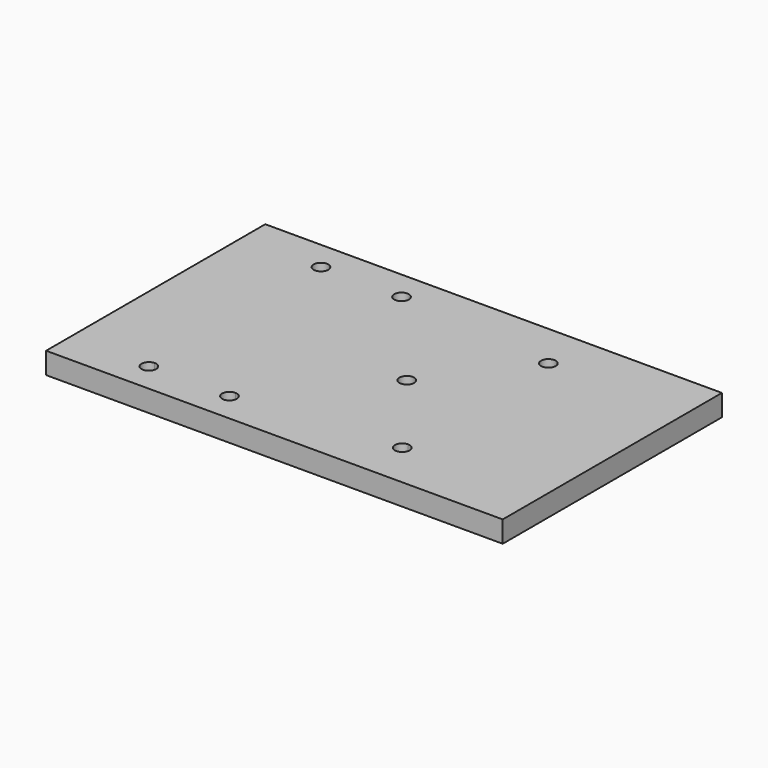
from build123d import *

# Parameters (mm, degrees)
F0_W     = 127
F0_H     = 76.2
F2_DEPTH = 5.969
F3_R     = 2.032
F4_DEPTH = 5.969


# Not quite as in the source:
# - a variable given as a bare number and used for a length is read in inches; the dataset says mm whatever the document's units were


with BuildPart() as f2:
    # F0 (on Top) → F2 (new body)
    with BuildSketch(Plane.XY):
        Rectangle(F0_W, F0_H)
    extrude(amount=F2_DEPTH)

    # F3 (on face) → F4 (cut, through all)
    with BuildSketch(Plane.XY.offset(5.969)):
        with BuildLine():
            ThreePointArc((-39.4335, -29.9085), (-40.0286590206, -28.4716590206), (-41.4655, -27.8765))
            ThreePointArc((-41.4655, -27.8765), (-42.9023409794, -31.3453409794), (-39.4335, -29.9085))
        make_face()
        with BuildLine():
            ThreePointArc((-17.018, -29.9085), (-17.6131590206, -28.4716590206), (-19.05, -27.8765))
            ThreePointArc((-19.05, -27.8765), (-20.4868409794, -31.3453409794), (-17.018, -29.9085))
        make_face()
        with BuildLine():
            Line((6.35, 0), (4.318, 0))
            ThreePointArc((4.318, 0), (6.35, -2.032), (8.382, 0))
            Line((8.382, 0), (6.35, 0))
        make_face()
        with BuildLine():
            ThreePointArc((8.382, 0), (6.35, 2.032), (4.318, 0))
            Line((4.318, 0), (6.35, 0))
            Line((6.35, 0), (8.382, 0))
        make_face()
        with BuildLine():
            ThreePointArc((27.432, -25.4), (26.8368409794, -23.9631590206), (25.4, -23.368))
            ThreePointArc((25.4, -23.368), (23.9631590206, -26.8368409794), (27.432, -25.4))
        make_face()
        with Locations((-41.4655, 29.9085)):
            Circle(F3_R)
        with Locations((-19.05, 29.9085)):
            Circle(F3_R)
        with Locations((25.4, 25.4)):
            Circle(F3_R)
    extrude(amount=-F4_DEPTH, mode=Mode.SUBTRACT)


solid = f2.part
